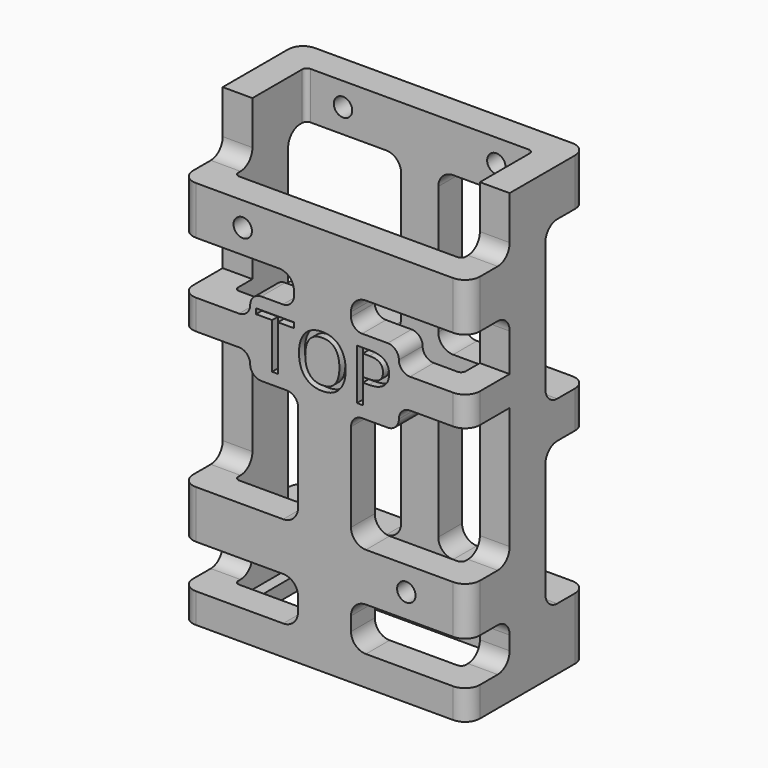
from build123d import *

# Parameters (mm, degrees)
F0_W         = 98.044
F0_H         = 50.8
F0_W_2       = 77.724
F0_H_2       = 30.48
F1_DEPTH     = 152.908
F2_R         = 3.1496
F3_DEPTH     = 10.16
F4_TEXT_SIZE = 24.2568471721
F5_DEPTH     = 2.54
F6_R         = 3.1496
F7_DEPTH     = 10.16
F8_W         = 77.724
F8_H         = 30.48
F8_W_2       = 70.104
F8_H_2       = 22.86
F9_DEPTH     = 5.08
F10_R        = 1.5875
F11_W        = 39.97325
F11_H        = 14.8844
F12_DEPTH    = 17.78
F13_W        = 42.672
F13_H        = 48.9204
F13_H_2      = 54.0004
F14_DEPTH    = 17.78
F15_R        = 5.08


# Not quite as in the source:
# - a feature names something its author has since deleted; it is built from what else it names
# - Text() gives the source's letters only with a copy of the font that has no kerning and outlines rounded to 1/6400 em; it was checked with that copy


with BuildPart() as f1:
    # F0 (on Top) → F1 (new body)
    with BuildSketch(Plane.XY):
        Rectangle(F0_W, F0_H)
        Rectangle(F0_W_2, F0_H_2, mode=Mode.SUBTRACT)
    extrude(amount=F1_DEPTH)

    # F2 (on face) → F3 (cut, through all)
    with BuildSketch(Plane.XZ.offset(25.4)):
        with Locations((-27.94, 124.714)):
            Circle(F2_R)
        with Locations((27.94, 33.274)):
            Circle(F2_R)
    extrude(amount=-F3_DEPTH, mode=Mode.SUBTRACT)

    # F4 (on face) → F5 (cut)
    with BuildSketch(Plane.XZ.offset(25.4)):
        with Locations((-23.622, 84.6430700361)):
            Text('TOP', F4_TEXT_SIZE, font='Open Sans', text_align=(TextAlign.LEFT, TextAlign.BOTTOM))
    extrude(amount=-F5_DEPTH, mode=Mode.SUBTRACT)

    # F6 (on face) → F7 (cut, through all)
    with BuildSketch(Plane(origin=(0, 25.4, 0), x_dir=(-1, 0, 0), z_dir=(0, 1, 0))):
        with Locations((26.2001, 145.034)):
            Circle(F6_R)
        with Locations((26.2001, 12.954)):
            Circle(F6_R)
        with Locations((-26.2001, 145.034)):
            Circle(F6_R)
        with Locations((-26.2001, 12.954)):
            Circle(F6_R)
    extrude(amount=-F7_DEPTH, mode=Mode.SUBTRACT)

    # F8 (on face) → F9 (join)
    with BuildSketch(Plane(origin=(0, 0, 0), x_dir=(1, 0, 0), z_dir=(0, 0, -1))):
        Rectangle(F8_W, F8_H)
        Rectangle(F8_W_2, F8_H_2, mode=Mode.SUBTRACT)
    extrude(amount=-F9_DEPTH)

    # F10
    f10_edges = [f1.edges().sort_by_distance(p)[0] for p in [
        (-38.862, 15.24, 78.994),
        (-38.862, -15.24, 78.994),
        (38.862, -15.24, 78.994),
        (38.862, 15.24, 78.994),
    ]]
    fillet(f10_edges, radius=F10_R)

    # F11 (on face) → F12 (cut)
    with BuildSketch(Plane.XZ.offset(25.4)):
        with Locations((29.035375, 17.6022)):
            Rectangle(F11_W, F11_H)
        with BuildLine():
            Line((9.04875, 41.5036), (49.022, 41.5036))
            Line((49.022, 41.5036), (49.022, 88.3029215552))
            Line((49.022, 88.3029215552), (29.21, 88.3029215552))
            ThreePointArc((29.21, 88.3029215552), (26.5159231637, 87.1869983916), (25.4, 84.4929215552))
            Line((25.4, 84.4929215552), (25.4, 84.4802215552))
            ThreePointArc((25.4, 84.4802215552), (24.2840768363, 81.7861447189), (21.59, 80.6702215552))
            Line((21.59, 80.6702215552), (12.85875, 80.6702215552))
            ThreePointArc((12.85875, 80.6702215552), (10.1646731637, 79.5542983916), (9.04875, 76.8602215552))
            Line((9.04875, 76.8602215552), (9.04875, 41.5036))
        make_face()
        with Locations((-29.035375, 17.6022)):
            Rectangle(F11_W, F11_H)
        with BuildLine():
            Line((-10.4285492178, 116.4844), (-49.022, 116.4844))
            Line((-49.022, 116.4844), (-49.022, 98.4629215552))
            Line((-49.022, 98.4629215552), (-29.21, 98.4629215552))
            ThreePointArc((-29.21, 98.4629215552), (-26.5159231637, 99.5788447189), (-25.4, 102.2729215552))
            Line((-25.4, 102.2729215552), (-25.4, 102.2856215552))
            ThreePointArc((-25.4, 102.2856215552), (-24.2840768363, 104.9796983916), (-21.59, 106.0956215552))
            Line((-21.59, 106.0956215552), (-14.2385492178, 106.0956215552))
            ThreePointArc((-14.2385492178, 106.0956215552), (-11.5444723815, 107.2115447189), (-10.4285492178, 109.9056215552))
            Line((-10.4285492178, 109.9056215552), (-10.4285492178, 116.4844))
        make_face()
        Polygon((-49.022, 152.908), (-49.022, 132.9436), (9.04875, 132.9436), (49.022, 132.9436), (49.022, 152.908), align=None)
        with BuildLine():
            Line((-49.022, 41.5036), (-9.04875, 41.5036))
            Line((-9.04875, 41.5036), (-9.04875, 76.8602215552))
            ThreePointArc((-9.04875, 76.8602215552), (-10.1646731637, 79.5542983916), (-12.85875, 80.6702215552))
            Line((-12.85875, 80.6702215552), (-21.59, 80.6702215552))
            ThreePointArc((-21.59, 80.6702215552), (-24.2840768363, 81.7861447189), (-25.4, 84.4802215552))
            Line((-25.4, 84.4802215552), (-25.4, 84.4929215552))
            ThreePointArc((-25.4, 84.4929215552), (-26.5159231637, 87.1869983916), (-29.21, 88.3029215552))
            Line((-29.21, 88.3029215552), (-49.022, 88.3029215552))
            Line((-49.022, 88.3029215552), (-49.022, 41.5036))
        make_face()
        with BuildLine():
            Line((9.04875, 116.4844), (9.04875, 109.9056215552))
            ThreePointArc((9.04875, 109.9056215552), (10.1646731637, 107.2115447189), (12.85875, 106.0956215552))
            Line((12.85875, 106.0956215552), (21.59, 106.0956215552))
            ThreePointArc((21.59, 106.0956215552), (24.2840768363, 104.9796983916), (25.4, 102.2856215552))
            ThreePointArc((25.4, 102.2856215552), (26.5159231637, 99.5915447189), (29.21, 98.4756215552))
            Line((29.21, 98.4756215552), (49.022, 98.4756215552))
            Line((49.022, 98.4756215552), (49.022, 116.4844))
            Line((49.022, 116.4844), (9.04875, 116.4844))
        make_face()
    extrude(amount=-F12_DEPTH, mode=Mode.SUBTRACT)

    # F13 (on face) → F14 (cut)
    with BuildSketch(Plane(origin=(0, 25.4, 0), x_dir=(-1, 0, 0), z_dir=(0, 1, 0))):
        with Locations((27.686, 45.6438)):
            Rectangle(F13_W, F13_H)
        with Locations((27.686, 109.8042)):
            Rectangle(F13_W, F13_H_2)
        with Locations((-27.686, 45.6438)):
            Rectangle(F13_W, F13_H)
        with Locations((-27.686, 109.8042)):
            Rectangle(F13_W, F13_H_2)
    extrude(amount=-F14_DEPTH, mode=Mode.SUBTRACT)

    # F15
    f15_edges = [f1.edges().sort_by_distance(p)[0] for p in [
        (43.942, -7.62, 10.16),
        (9.04875, -20.32, 10.16),
        (9.04875, -20.32, 25.0444),
        (43.942, -7.62, 25.0444),
        (-9.04875, -20.32, 10.16),
        (-9.04875, -20.32, 25.0444),
        (-43.942, -7.62, 25.0444),
        (-43.942, -7.62, 10.16),
        (-43.942, -7.62, 41.5036),
        (-9.04875, -20.32, 41.5036),
        (43.942, -7.62, 41.5036),
        (9.04875, -20.32, 41.5036),
        (-43.942, -7.62, 116.4844),
        (-10.428549, -20.32, 116.4844),
        (9.04875, -20.32, 116.4844),
        (43.942, -7.62, 116.4844),
        (-43.942, -7.62, 132.9436),
        (43.942, -7.62, 132.9436),
        (-43.942, 7.62, 70.104),
        (-43.942, 7.62, 82.804),
        (-43.942, 7.62, 21.1836),
        (-6.35, 20.32, 21.1836),
        (-6.35, 20.32, 70.104),
        (-6.35, 20.32, 82.804),
        (-43.942, 7.62, 136.8044),
        (-6.35, 20.32, 136.8044),
        (6.35, 20.32, 136.8044),
        (43.942, 7.62, 136.8044),
        (6.35, 20.32, 82.804),
        (43.942, 7.62, 82.804),
        (6.35, 20.32, 21.1836),
        (6.35, 20.32, 70.104),
        (43.942, 7.62, 70.104),
        (43.942, 7.62, 21.1836),
        (49.022, -25.4, 124.714),
        (49.022, -25.4, 33.274),
        (49.022, -25.4, 5.08),
        (49.022, 25.4, 10.5918),
        (49.022, 25.4, 76.454),
        (49.022, 25.4, 144.8562),
        (-49.022, 25.4, 144.8562),
        (-49.022, 25.4, 76.454),
        (-49.022, 25.4, 10.5918),
        (-49.022, -25.4, 5.08),
        (-49.022, -25.4, 33.274),
        (-49.022, -25.4, 124.714),
        (35.052, -11.43, 2.54),
        (35.052, 11.43, 2.54),
        (-35.052, -11.43, 2.54),
        (-35.052, 11.43, 2.54),
        (49.022, -25.4, 93.389272),
        (-49.022, -25.4, 93.382922),
    ]]
    fillet(f15_edges, radius=F15_R)


solid = f1.part
